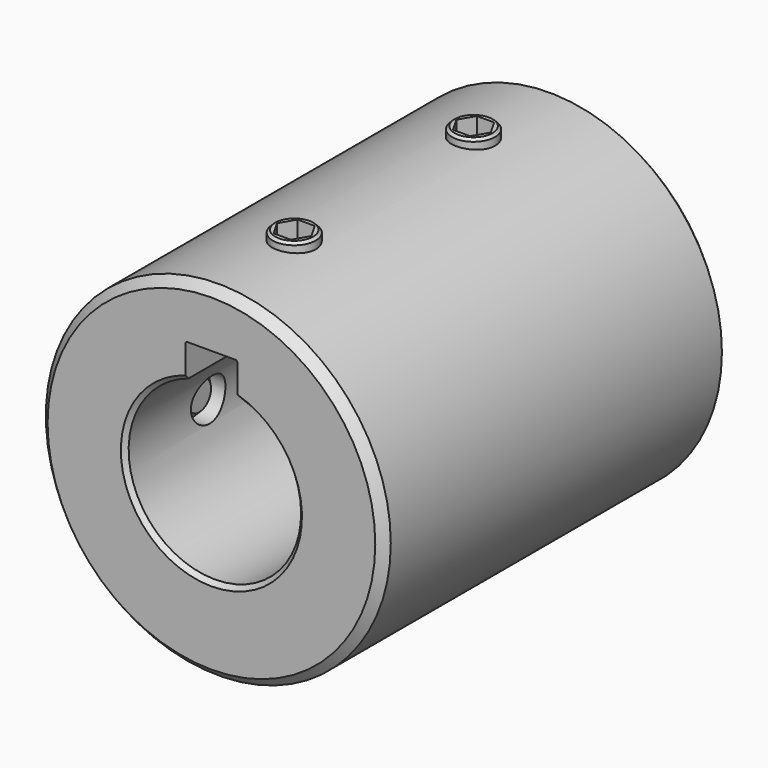
from build123d import *

# Parameters (mm, degrees)
F0_R         = 20
F1_DEPTH     = 50
F2_SIZE      = 1
F3_R         = 2.5
F4_DEPTH     = 6.4616079858
F6_R         = 2.5
F7_DEPTH     = 20.0010001
F8_START     = -11
F8_DEPTH     = 10
F9_START     = -1
F9_DEPTH     = 6.5
F10_SIZE     = 0.8
F10_2_SIZE   = 0.8
F10_3_SIZE   = 0.8
F10_4_SIZE   = 0.8
F12_DEPTH    = 3
F13_SIZE     = 0.3
F13_2_SIZE   = 0.3
F13_3_SIZE   = 0.3
F13_4_SIZE   = 0.3
F15_DEPTH    = 3
F16_T2_ANGLE = 338.6533053812
F16_T4_ANGLE = 338.6533053812


# Not quite as in the source:
# - a fillet or chamfer that OpenCascade refuses, or shapes differently, is made with other operations: its cross-section is extruded or revolved along the edge and cut away or added
# - a feature names something its author has since deleted; it is built from what else it names


with BuildPart() as f1:
    # F0 (on Front) → F1 (new body)
    with BuildSketch(Plane.XZ):
        with Locations((-120.1100092272, 70.6079402205)):
            Circle(F0_R)
        with BuildLine():
            ThreePointArc((-123.1100092272, 83.9473322347), (-123.0514305834, 84.0887535909), (-122.9100092272, 84.1473322347))
            Line((-122.9100092272, 84.1473322347), (-117.3100092272, 84.1473322347))
            ThreePointArc((-117.3100092272, 84.1473322347), (-117.168587871, 84.0887535909), (-117.1100092272, 83.9473322347))
            Line((-117.1100092272, 83.9473322347), (-117.1100092272, 80.2929802308))
            ThreePointArc((-117.1100092272, 80.2929802308), (-117.0721033659, 80.1758243935), (-116.9727543252, 80.1030774855))
            ThreePointArc((-116.9727543252, 80.1030774855), (-120.1457476597, 60.6080040825), (-123.1793161579, 80.1252589062))
            ThreePointArc((-123.1793161579, 80.1252589062), (-123.1291720237, 80.161564899), (-123.1100092272, 80.2204320931))
            Line((-123.1100092272, 80.2204320931), (-123.1100092272, 83.9473322347))
        make_face(mode=Mode.SUBTRACT)
    extrude(amount=-F1_DEPTH)

    # F2
    f2_edges = [f1.edges().sort_by_distance(p)[0] for p in [
        (-140.110009, 0, 70.60794),
        (-140.110009, 50, 70.60794),
    ]]
    chamfer(f2_edges, length=F2_SIZE)

    # F3 (on face) → F4 (cut, through all)
    with BuildSketch(Plane(origin=(0, 0, 84.1473322347), x_dir=(1, 0, 0), z_dir=(0, 0, -1))):
        with Locations((-120.1100092272, -12)):
            Circle(F3_R)
        with Locations((-120.1100092272, -38)):
            Circle(F3_R)
    extrude(amount=-F4_DEPTH, mode=Mode.SUBTRACT)

    # F6 (on offset) → F7 (cut, through all)
    with BuildSketch(Plane.YZ.offset(-120.1100092272)):
        with Locations((12, 71.1473322347)):
            Circle(F6_R)
        with Locations((38, 71.1473322347)):
            Circle(F6_R)
    extrude(amount=-F7_DEPTH, mode=Mode.SUBTRACT)

    # F16: chamfer of 0.5 on 2 edges, made by hand

    # F16_s1 → F16_t2 (revolve, cut)
    with BuildSketch(Plane(origin=(-128.9179601882, 0, 24.7746190281), x_dir=(0, 1, 0), z_dir=(-0.9820308726, 0, 0.1887203358))):
        Polygon((0, -57.1719758706), (0.5, -56.6719758706), (0, -56.6719758706), align=None)
    revolve(axis=Axis((-120.1100092272, 0, 70.6079402205), (0, 1, 0)), revolution_arc=F16_T2_ANGLE, mode=Mode.SUBTRACT)

    # F16_s3 → F16_t4 (revolve, cut)
    with BuildSketch(Plane(origin=(-128.9179601882, 0, 24.7746190281), x_dir=(0, 1, 0), z_dir=(-0.9820308726, 0, 0.1887203358))):
        Polygon((50, -57.1719758706), (49.5, -56.6719758706), (50, -56.6719758706), align=None)
    revolve(axis=Axis((-120.1100092272, 50, 70.6079402205), (0, 1, 0)), revolution_arc=F16_T4_ANGLE, mode=Mode.SUBTRACT)


with BuildPart() as f8:
    # F6 (on offset) → F8 (new body)
    with BuildSketch(Plane.YZ.offset(-120.1100092272).offset(F8_START)):
        with Locations((38, 71.1473322347)):
            Circle(F6_R)
    extrude(amount=-F8_DEPTH)

    # F10
    f10_edges = [f8.edges().sort_by_distance(p)[0] for p in [
        (-131.110009, 35.5, 71.147332),
    ]]
    chamfer(f10_edges, length=F10_SIZE)

    # F13
    f13_edges = [f8.edges().sort_by_distance(p)[0] for p in [
        (-141.110009, 35.5, 71.147332),
    ]]
    chamfer(f13_edges, length=F13_SIZE)


with BuildPart() as f8b:
    # F6 (on offset) → F8, piece 2 (new body)
    with BuildSketch(Plane.YZ.offset(-120.1100092272).offset(F8_START)):
        with Locations((12, 71.1473322347)):
            Circle(F6_R)
    extrude(amount=-F8_DEPTH)

    # F10#2
    f10_2_edges = [f8b.edges().sort_by_distance(p)[0] for p in [
        (-131.110009, 9.5, 71.147332),
    ]]
    chamfer(f10_2_edges, length=F10_2_SIZE)

    # F13#2
    f13_2_edges = [f8b.edges().sort_by_distance(p)[0] for p in [
        (-141.110009, 9.5, 71.147332),
    ]]
    chamfer(f13_2_edges, length=F13_2_SIZE)


with BuildPart() as f9:
    # F3 (on face) → F9 (new body)
    with BuildSketch(Plane(origin=(0, 0, 84.1473322347), x_dir=(1, 0, 0), z_dir=(0, 0, -1)).offset(F9_START)):
        with Locations((-120.1100092272, -38)):
            Circle(F3_R)
    extrude(amount=-F9_DEPTH)

    # F10#3
    f10_3_edges = [f9.edges().sort_by_distance(p)[0] for p in [
        (-122.610009, 38, 85.147332),
    ]]
    chamfer(f10_3_edges, length=F10_3_SIZE)


with BuildPart() as f9b:
    # F3 (on face) → F9, piece 2 (new body)
    with BuildSketch(Plane(origin=(0, 0, 84.1473322347), x_dir=(1, 0, 0), z_dir=(0, 0, -1)).offset(F9_START)):
        with Locations((-120.1100092272, -12)):
            Circle(F3_R)
    extrude(amount=-F9_DEPTH)

    # F10#4
    f10_4_edges = [f9b.edges().sort_by_distance(p)[0] for p in [
        (-122.610009, 12, 85.147332),
    ]]
    chamfer(f10_4_edges, length=F10_4_SIZE)


with BuildPart() as f12_tool:
    # F11 (on face) → F12 (new body)
    with BuildSketch(Plane.XY.offset(91.6473322347)):
        Polygon((-121.1100092272, 36.2679491924), (-119.1100092272, 36.2679491924), (-118.1100092272, 38), (-119.1100092272, 39.7320508076), (-121.1100092272, 39.7320508076), (-122.1100092272, 38), align=None)
        Polygon((-121.1100092272, 10.2679491924), (-119.1100092272, 10.2679491924), (-118.1100092272, 12), (-119.1100092272, 13.7320508076), (-121.1100092272, 13.7320508076), (-122.1100092272, 12), align=None)
    extrude(amount=-F12_DEPTH)


with BuildPart() as f9_1:
    add(f9.part)

    # F12: cut by f12_tool
    add(f12_tool.part, mode=Mode.SUBTRACT)

    # F13#3
    f13_3_edges = [f9_1.edges().sort_by_distance(p)[0] for p in [
        (-122.610009, 38, 91.647332),
    ]]
    chamfer(f13_3_edges, length=F13_3_SIZE)


with BuildPart() as f9b_1:
    add(f9b.part)

    # F12: cut by f12_tool
    add(f12_tool.part, mode=Mode.SUBTRACT)

    # F13#4
    f13_4_edges = [f9b_1.edges().sort_by_distance(p)[0] for p in [
        (-122.610009, 12, 91.647332),
    ]]
    chamfer(f13_4_edges, length=F13_4_SIZE)


with BuildPart() as f15_tool:
    # F14 (on face) → F15 (new body)
    with BuildSketch(Plane(origin=(-141.1100092272, 0, 0), x_dir=(0, -1, 0), z_dir=(-1, 0, 0))):
        Polygon((-39, 69.4152814271), (-37, 69.4152814271), (-36, 71.1473322347), (-37, 72.8793830423), (-39, 72.8793830423), (-40, 71.1473322347), align=None)
        Polygon((-13, 69.4152814271), (-11, 69.4152814271), (-10, 71.1473322347), (-11, 72.8793830423), (-13, 72.8793830423), (-14, 71.1473322347), align=None)
    extrude(amount=-F15_DEPTH)


with BuildPart() as f8_1:
    add(f8.part)

    # F15: cut by f15_tool
    add(f15_tool.part, mode=Mode.SUBTRACT)


with BuildPart() as f8b_1:
    add(f8b.part)

    # F15: cut by f15_tool
    add(f15_tool.part, mode=Mode.SUBTRACT)


solid = Compound([f1.part, f9_1.part, f9b_1.part, f8_1.part, f8b_1.part])
